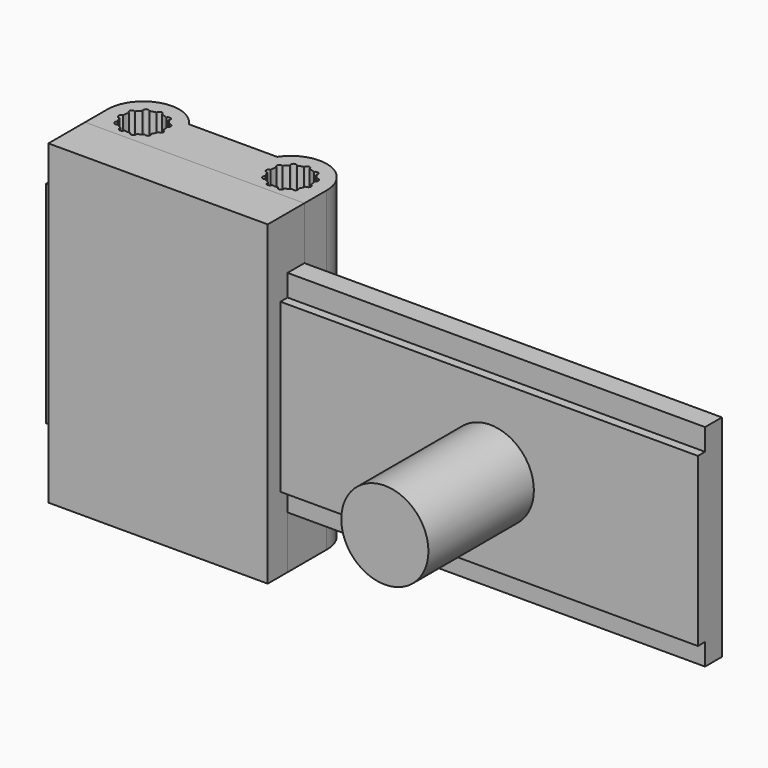
from build123d import *

# Parameters (mm, degrees)
F2_DEPTH       = 25
F2_DEPTH_BACK  = 100
F3_START       = 14
F1_W           = 1.190625
F1_H           = 31.75
F1_W_2         = 0.5
F3_DEPTH       = 86
F4_R           = 4.55
F5_DEPTH       = 30
F5_DEPTH_BACK  = 30
F6_DEPTH       = 15
F6_DEPTH_BACK  = 15
F7_W           = 41.6
F7_H           = 10
F8_DEPTH       = 4
F9_W           = 41.6
F9_H           = 4.690625
F10_DEPTH      = 30
F10_DEPTH_BACK = 30
F11_DEPTH      = 4
F12_START      = 14
F12_DEPTH      = 11
F13_R          = 8.2657207396
F14_DEPTH      = 25


# Not quite as in the source:
# - a feature names something its author has since deleted; it is built from what else it names


with BuildPart() as f2:
    # F1 (on Right) → F2 (new body, two sides)
    with BuildSketch(Plane.YZ) as f2_sk:
        Polygon((2, -20), (2, 20), (-2, 20), (-2, 15.875), (-2, -15.875), (-2, -20), align=None)
    extrude(amount=-F2_DEPTH)
    extrude(f2_sk.sketch, amount=F2_DEPTH_BACK)

    # F1 (on Right) → F3 (join)
    with BuildSketch(Plane.YZ.offset(F3_START)):
        with Locations((-3.0953125, 0)):
            Rectangle(F1_W, F1_H)
        with Locations((-2.25, 0)):
            Rectangle(F1_W_2, F1_H)
    extrude(amount=F3_DEPTH)

    # F13 (on face) → F14 (join)
    with BuildSketch(Plane.XZ.offset(3.690625)):
        with Locations((60.6145299971, 0)):
            Circle(F13_R)
    extrude(amount=F14_DEPTH)


with BuildPart() as f5:
    # F4 (on Top) → F5 (new body, two sides)
    with BuildSketch(Plane.XY) as f5_sk:
        with BuildLine():
            Line((-20.8, 2), (-9.7397183192, 2))
            ThreePointArc((-9.7397183192, 2), (-7.2767432507, 6.2812661375), (-8.3608511281, 11.1))
            ThreePointArc((-8.3608511281, 11.1), (-15.9866790972, 13.8033150135), (-20.8, 7.3))
            Line((-20.8, 7.3), (-20.8, 2))
        make_face()
        with Locations((-14, 7.3)):
            Circle(F4_R, mode=Mode.SUBTRACT)
        with Locations((-14, 7.3)):
            Circle(F4_R)
        with BuildLine():
            ThreePointArc((-17.2194219637, 9.3187427324), (-16.8718483825, 9.788470789), (-16.4563663583, 10.1993558446))
            ThreePointArc((-16.4563663583, 10.1993558446), (-16.3247555151, 10.9173901912), (-15.6169353795, 10.7388253777))
            ThreePointArc((-15.6169353795, 10.7388253777), (-15.070583716, 10.9460732997), (-14.4989167629, 11.0671052632))
            ThreePointArc((-14.4989167629, 11.0671052632), (-14, 11.6), (-13.5010832371, 11.0671052632))
            ThreePointArc((-13.5010832371, 11.0671052632), (-12.929416284, 10.9460732997), (-12.3830646205, 10.7388253777))
            ThreePointArc((-12.3830646205, 10.7388253777), (-11.6752444849, 10.9173901912), (-11.5436336417, 10.1993558446))
            ThreePointArc((-11.5436336417, 10.1993558446), (-11.1281516175, 9.788470789), (-10.7805780363, 9.3187427324))
            ThreePointArc((-10.7805780363, 9.3187427324), (-10.08858242, 9.0862845559), (-10.3660630092, 8.4110814313))
            ThreePointArc((-10.3660630092, 8.4110814313), (-10.2386785209, 7.8407963854), (-10.2002351783, 7.2577235333))
            ThreePointArc((-10.2002351783, 7.2577235333), (-9.7437677999, 6.6880461954), (-10.3422416951, 6.2700465141))
            ThreePointArc((-10.3422416951, 6.2700465141), (-10.5433984177, 5.7214229506), (-10.8262908033, 5.2101268137))
            ThreePointArc((-10.8262908033, 5.2101268137), (-10.7502768303, 4.484098844), (-11.4797327983, 4.4560145513))
            ThreePointArc((-11.4797327983, 4.4560145513), (-11.9455648937, 4.1032365752), (-12.4599766739, 3.8260500644))
            ThreePointArc((-12.4599766739, 3.8260500644), (-12.7885500056, 3.1741802135), (-13.4173909307, 3.5449278739))
            ThreePointArc((-13.4173909307, 3.5449278739), (-14, 3.5), (-14.5826090693, 3.5449278739))
            ThreePointArc((-14.5826090693, 3.5449278739), (-15.2114499944, 3.1741802135), (-15.5400233261, 3.8260500644))
            ThreePointArc((-15.5400233261, 3.8260500644), (-16.0544351063, 4.1032365752), (-16.5202672017, 4.4560145513))
            ThreePointArc((-16.5202672017, 4.4560145513), (-17.2497231697, 4.484098844), (-17.1737091967, 5.2101268137))
            ThreePointArc((-17.1737091967, 5.2101268137), (-17.4566015823, 5.7214229506), (-17.6577583049, 6.2700465141))
            ThreePointArc((-17.6577583049, 6.2700465141), (-18.2562322001, 6.6880461954), (-17.7997648217, 7.2577235333))
            ThreePointArc((-17.7997648217, 7.2577235333), (-17.7613214791, 7.8407963854), (-17.6339369908, 8.4110814313))
            ThreePointArc((-17.6339369908, 8.4110814313), (-17.91141758, 9.0862845559), (-17.2194219637, 9.3187427324))
        make_face(mode=Mode.SUBTRACT)
        with BuildLine():
            ThreePointArc((-8.3608511281, 11.1), (-7.2767432507, 6.2812661375), (-9.7397183192, 2))
            Line((-9.7397183192, 2), (9.7397183192, 2))
            ThreePointArc((9.7397183192, 2), (7.2767432507, 6.2812661375), (8.3608511281, 11.1))
            Line((8.3608511281, 11.1), (-8.3608511281, 11.1))
        make_face()
        with BuildLine():
            ThreePointArc((8.3608511281, 11.1), (7.2767432507, 6.2812661375), (9.7397183192, 2))
            Line((9.7397183192, 2), (20.8, 2))
            Line((20.8, 2), (20.8, 7.3))
            ThreePointArc((20.8, 7.3), (15.9866790972, 13.8033150135), (8.3608511281, 11.1))
        make_face()
        with Locations((14, 7.3)):
            Circle(F4_R, mode=Mode.SUBTRACT)
        with Locations((14, 7.3)):
            Circle(F4_R)
        with BuildLine():
            ThreePointArc((12.3830646205, 10.7388253777), (12.929416284, 10.9460732997), (13.5010832371, 11.0671052632))
            ThreePointArc((13.5010832371, 11.0671052632), (14, 11.6), (14.4989167629, 11.0671052632))
            ThreePointArc((14.4989167629, 11.0671052632), (15.070583716, 10.9460732997), (15.6169353795, 10.7388253777))
            ThreePointArc((15.6169353795, 10.7388253777), (16.3247555151, 10.9173901912), (16.4563663583, 10.1993558446))
            ThreePointArc((16.4563663583, 10.1993558446), (16.8718483825, 9.788470789), (17.2194219637, 9.3187427324))
            ThreePointArc((17.2194219637, 9.3187427324), (17.91141758, 9.0862845559), (17.6339369908, 8.4110814313))
            ThreePointArc((17.6339369908, 8.4110814313), (17.7613214791, 7.8407963854), (17.7997648217, 7.2577235333))
            ThreePointArc((17.7997648217, 7.2577235333), (18.2562322001, 6.6880461954), (17.6577583049, 6.2700465141))
            ThreePointArc((17.6577583049, 6.2700465141), (17.4566015823, 5.7214229506), (17.1737091967, 5.2101268137))
            ThreePointArc((17.1737091967, 5.2101268137), (17.2497231697, 4.484098844), (16.5202672017, 4.4560145513))
            ThreePointArc((16.5202672017, 4.4560145513), (16.0544351063, 4.1032365752), (15.5400233261, 3.8260500644))
            ThreePointArc((15.5400233261, 3.8260500644), (15.2114499944, 3.1741802135), (14.5826090693, 3.5449278739))
            ThreePointArc((14.5826090693, 3.5449278739), (14, 3.5), (13.4173909307, 3.5449278739))
            ThreePointArc((13.4173909307, 3.5449278739), (12.7885500056, 3.1741802135), (12.4599766739, 3.8260500644))
            ThreePointArc((12.4599766739, 3.8260500644), (11.9455648937, 4.1032365752), (11.4797327983, 4.4560145513))
            ThreePointArc((11.4797327983, 4.4560145513), (10.7502768303, 4.484098844), (10.8262908033, 5.2101268137))
            ThreePointArc((10.8262908033, 5.2101268137), (10.5433984177, 5.7214229506), (10.3422416951, 6.2700465141))
            ThreePointArc((10.3422416951, 6.2700465141), (9.7437677999, 6.6880461954), (10.2002351783, 7.2577235333))
            ThreePointArc((10.2002351783, 7.2577235333), (10.2386785209, 7.8407963854), (10.3660630092, 8.4110814313))
            ThreePointArc((10.3660630092, 8.4110814313), (10.08858242, 9.0862845559), (10.7805780363, 9.3187427324))
            ThreePointArc((10.7805780363, 9.3187427324), (11.1281516175, 9.788470789), (11.5436336417, 10.1993558446))
            ThreePointArc((11.5436336417, 10.1993558446), (11.6752444849, 10.9173901912), (12.3830646205, 10.7388253777))
        make_face(mode=Mode.SUBTRACT)
    extrude(amount=-F5_DEPTH)
    extrude(f5_sk.sketch, amount=F5_DEPTH_BACK)

    # F4 (on Top) → F6 (cut, two sides)
    with BuildSketch(Plane.XY) as f6_sk:
        with Locations((-14, 7.3)):
            Circle(F4_R)
        with BuildLine():
            ThreePointArc((-17.2194219637, 9.3187427324), (-16.8718483825, 9.788470789), (-16.4563663583, 10.1993558446))
            ThreePointArc((-16.4563663583, 10.1993558446), (-16.3247555151, 10.9173901912), (-15.6169353795, 10.7388253777))
            ThreePointArc((-15.6169353795, 10.7388253777), (-15.070583716, 10.9460732997), (-14.4989167629, 11.0671052632))
            ThreePointArc((-14.4989167629, 11.0671052632), (-14, 11.6), (-13.5010832371, 11.0671052632))
            ThreePointArc((-13.5010832371, 11.0671052632), (-12.929416284, 10.9460732997), (-12.3830646205, 10.7388253777))
            ThreePointArc((-12.3830646205, 10.7388253777), (-11.6752444849, 10.9173901912), (-11.5436336417, 10.1993558446))
            ThreePointArc((-11.5436336417, 10.1993558446), (-11.1281516175, 9.788470789), (-10.7805780363, 9.3187427324))
            ThreePointArc((-10.7805780363, 9.3187427324), (-10.08858242, 9.0862845559), (-10.3660630092, 8.4110814313))
            ThreePointArc((-10.3660630092, 8.4110814313), (-10.2386785209, 7.8407963854), (-10.2002351783, 7.2577235333))
            ThreePointArc((-10.2002351783, 7.2577235333), (-9.7437677999, 6.6880461954), (-10.3422416951, 6.2700465141))
            ThreePointArc((-10.3422416951, 6.2700465141), (-10.5433984177, 5.7214229506), (-10.8262908033, 5.2101268137))
            ThreePointArc((-10.8262908033, 5.2101268137), (-10.7502768303, 4.484098844), (-11.4797327983, 4.4560145513))
            ThreePointArc((-11.4797327983, 4.4560145513), (-11.9455648937, 4.1032365752), (-12.4599766739, 3.8260500644))
            ThreePointArc((-12.4599766739, 3.8260500644), (-12.7885500056, 3.1741802135), (-13.4173909307, 3.5449278739))
            ThreePointArc((-13.4173909307, 3.5449278739), (-14, 3.5), (-14.5826090693, 3.5449278739))
            ThreePointArc((-14.5826090693, 3.5449278739), (-15.2114499944, 3.1741802135), (-15.5400233261, 3.8260500644))
            ThreePointArc((-15.5400233261, 3.8260500644), (-16.0544351063, 4.1032365752), (-16.5202672017, 4.4560145513))
            ThreePointArc((-16.5202672017, 4.4560145513), (-17.2497231697, 4.484098844), (-17.1737091967, 5.2101268137))
            ThreePointArc((-17.1737091967, 5.2101268137), (-17.4566015823, 5.7214229506), (-17.6577583049, 6.2700465141))
            ThreePointArc((-17.6577583049, 6.2700465141), (-18.2562322001, 6.6880461954), (-17.7997648217, 7.2577235333))
            ThreePointArc((-17.7997648217, 7.2577235333), (-17.7613214791, 7.8407963854), (-17.6339369908, 8.4110814313))
            ThreePointArc((-17.6339369908, 8.4110814313), (-17.91141758, 9.0862845559), (-17.2194219637, 9.3187427324))
        make_face(mode=Mode.SUBTRACT)
        with Locations((14, 7.3)):
            Circle(F4_R)
        with BuildLine():
            ThreePointArc((12.3830646205, 10.7388253777), (12.929416284, 10.9460732997), (13.5010832371, 11.0671052632))
            ThreePointArc((13.5010832371, 11.0671052632), (14, 11.6), (14.4989167629, 11.0671052632))
            ThreePointArc((14.4989167629, 11.0671052632), (15.070583716, 10.9460732997), (15.6169353795, 10.7388253777))
            ThreePointArc((15.6169353795, 10.7388253777), (16.3247555151, 10.9173901912), (16.4563663583, 10.1993558446))
            ThreePointArc((16.4563663583, 10.1993558446), (16.8718483825, 9.788470789), (17.2194219637, 9.3187427324))
            ThreePointArc((17.2194219637, 9.3187427324), (17.91141758, 9.0862845559), (17.6339369908, 8.4110814313))
            ThreePointArc((17.6339369908, 8.4110814313), (17.7613214791, 7.8407963854), (17.7997648217, 7.2577235333))
            ThreePointArc((17.7997648217, 7.2577235333), (18.2562322001, 6.6880461954), (17.6577583049, 6.2700465141))
            ThreePointArc((17.6577583049, 6.2700465141), (17.4566015823, 5.7214229506), (17.1737091967, 5.2101268137))
            ThreePointArc((17.1737091967, 5.2101268137), (17.2497231697, 4.484098844), (16.5202672017, 4.4560145513))
            ThreePointArc((16.5202672017, 4.4560145513), (16.0544351063, 4.1032365752), (15.5400233261, 3.8260500644))
            ThreePointArc((15.5400233261, 3.8260500644), (15.2114499944, 3.1741802135), (14.5826090693, 3.5449278739))
            ThreePointArc((14.5826090693, 3.5449278739), (14, 3.5), (13.4173909307, 3.5449278739))
            ThreePointArc((13.4173909307, 3.5449278739), (12.7885500056, 3.1741802135), (12.4599766739, 3.8260500644))
            ThreePointArc((12.4599766739, 3.8260500644), (11.9455648937, 4.1032365752), (11.4797327983, 4.4560145513))
            ThreePointArc((11.4797327983, 4.4560145513), (10.7502768303, 4.484098844), (10.8262908033, 5.2101268137))
            ThreePointArc((10.8262908033, 5.2101268137), (10.5433984177, 5.7214229506), (10.3422416951, 6.2700465141))
            ThreePointArc((10.3422416951, 6.2700465141), (9.7437677999, 6.6880461954), (10.2002351783, 7.2577235333))
            ThreePointArc((10.2002351783, 7.2577235333), (10.2386785209, 7.8407963854), (10.3660630092, 8.4110814313))
            ThreePointArc((10.3660630092, 8.4110814313), (10.08858242, 9.0862845559), (10.7805780363, 9.3187427324))
            ThreePointArc((10.7805780363, 9.3187427324), (11.1281516175, 9.788470789), (11.5436336417, 10.1993558446))
            ThreePointArc((11.5436336417, 10.1993558446), (11.6752444849, 10.9173901912), (12.3830646205, 10.7388253777))
        make_face(mode=Mode.SUBTRACT)
        with BuildLine():
            ThreePointArc((14.4989167629, 11.0671052632), (14, 11.6), (13.5010832371, 11.0671052632))
            ThreePointArc((13.5010832371, 11.0671052632), (12.929416284, 10.9460732997), (12.3830646205, 10.7388253777))
            ThreePointArc((12.3830646205, 10.7388253777), (11.6752444849, 10.9173901912), (11.5436336417, 10.1993558446))
            ThreePointArc((11.5436336417, 10.1993558446), (11.1281516175, 9.788470789), (10.7805780363, 9.3187427324))
            ThreePointArc((10.7805780363, 9.3187427324), (10.08858242, 9.0862845559), (10.3660630092, 8.4110814313))
            ThreePointArc((10.3660630092, 8.4110814313), (10.2386785209, 7.8407963854), (10.2002351783, 7.2577235333))
            ThreePointArc((10.2002351783, 7.2577235333), (9.7437677999, 6.6880461954), (10.3422416951, 6.2700465141))
            ThreePointArc((10.3422416951, 6.2700465141), (10.5433984177, 5.7214229506), (10.8262908033, 5.2101268137))
            ThreePointArc((10.8262908033, 5.2101268137), (10.7502768303, 4.484098844), (11.4797327983, 4.4560145513))
            ThreePointArc((11.4797327983, 4.4560145513), (11.9455648937, 4.1032365752), (12.4599766739, 3.8260500644))
            ThreePointArc((12.4599766739, 3.8260500644), (12.7885500056, 3.1741802135), (13.4173909307, 3.5449278739))
            ThreePointArc((13.4173909307, 3.5449278739), (14, 3.5), (14.5826090693, 3.5449278739))
            ThreePointArc((14.5826090693, 3.5449278739), (15.2114499944, 3.1741802135), (15.5400233261, 3.8260500644))
            ThreePointArc((15.5400233261, 3.8260500644), (16.0544351063, 4.1032365752), (16.5202672017, 4.4560145513))
            ThreePointArc((16.5202672017, 4.4560145513), (17.2497231697, 4.484098844), (17.1737091967, 5.2101268137))
            ThreePointArc((17.1737091967, 5.2101268137), (17.4566015823, 5.7214229506), (17.6577583049, 6.2700465141))
            ThreePointArc((17.6577583049, 6.2700465141), (18.2562322001, 6.6880461954), (17.7997648217, 7.2577235333))
            ThreePointArc((17.7997648217, 7.2577235333), (17.7613214791, 7.8407963854), (17.6339369908, 8.4110814313))
            ThreePointArc((17.6339369908, 8.4110814313), (17.91141758, 9.0862845559), (17.2194219637, 9.3187427324))
            ThreePointArc((17.2194219637, 9.3187427324), (16.8718483825, 9.788470789), (16.4563663583, 10.1993558446))
            ThreePointArc((16.4563663583, 10.1993558446), (16.3247555151, 10.9173901912), (15.6169353795, 10.7388253777))
            ThreePointArc((15.6169353795, 10.7388253777), (15.070583716, 10.9460732997), (14.4989167629, 11.0671052632))
        make_face()
    extrude(amount=F6_DEPTH, mode=Mode.SUBTRACT)
    extrude(f6_sk.sketch, amount=-F6_DEPTH_BACK, mode=Mode.SUBTRACT)

    # F7 (on face) → F8 (join)
    with BuildSketch(Plane.XZ.offset(-2)):
        with Locations((0, -25)):
            Rectangle(F7_W, F7_H)
    extrude(amount=F8_DEPTH)


with BuildPart() as f10:
    # F9 (on Top) → F10 (new body, two sides)
    with BuildSketch(Plane.XY) as f10_sk:
        with Locations((0, -4.3453125)):
            Rectangle(F9_W, F9_H)
    extrude(amount=F10_DEPTH)
    extrude(f10_sk.sketch, amount=-F10_DEPTH_BACK)

    # F7 (on face) → F11 (join, through all)
    with BuildSketch(Plane.XZ.offset(-2)):
        with Locations((0, 25)):
            Rectangle(F7_W, F7_H)
    extrude(amount=F11_DEPTH)

    # F1 (on Right) → F12 (cut)
    with BuildSketch(Plane.YZ.offset(F12_START)):
        with Locations((-2.25, 0)):
            Rectangle(F1_W_2, F1_H)
        with Locations((-3.0953125, 0)):
            Rectangle(F1_W, F1_H)
    extrude(amount=F12_DEPTH, mode=Mode.SUBTRACT)


solid = Compound([f2.part, f5.part, f10.part])
